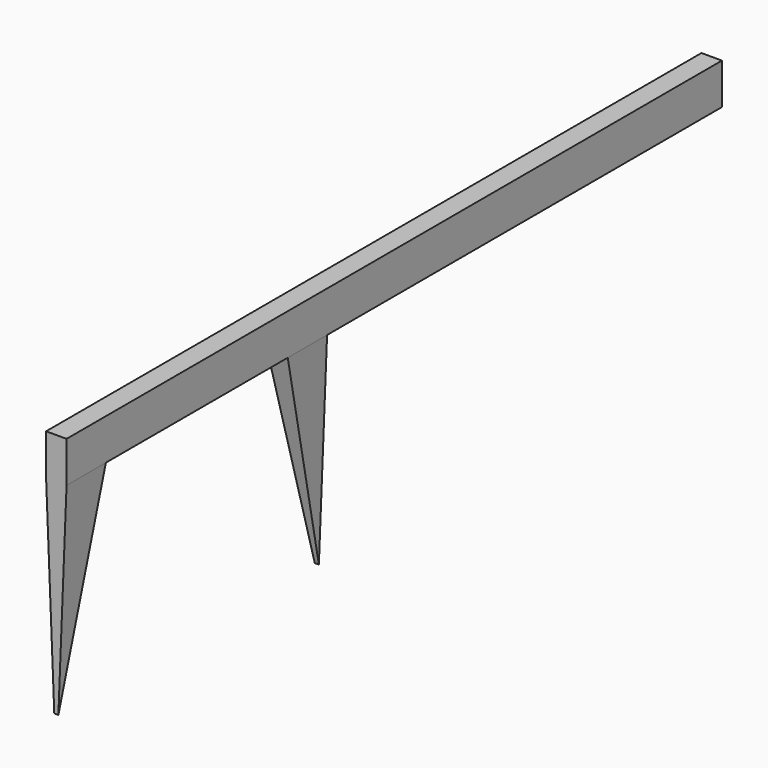
from build123d import *

# Parameters (mm, degrees)
F1_DEPTH = 5
F3_DEPTH = 200.001


# Not quite as in the source:
# - a feature names something its author has since deleted; it is built from what else it names


with BuildPart() as f1:
    # F0 (on Right) → F1 (new body)
    with BuildSketch(Plane.YZ):
        Polygon((200, 60), (0, 60), (0, 0), (12, 50), (67.5, 50), (79.5, 0), (79.5, 50), (200, 50), align=None)
    extrude(amount=F1_DEPTH)

    # F2 (on face) → F3 (cut, through all)
    with BuildSketch(Plane.XZ):
        Polygon((2, 0), (0, 50), (0, 0), align=None)
        Polygon((5, 0), (5, 50), (3, 0), align=None)
    extrude(amount=-F3_DEPTH, mode=Mode.SUBTRACT)


solid = f1.part
